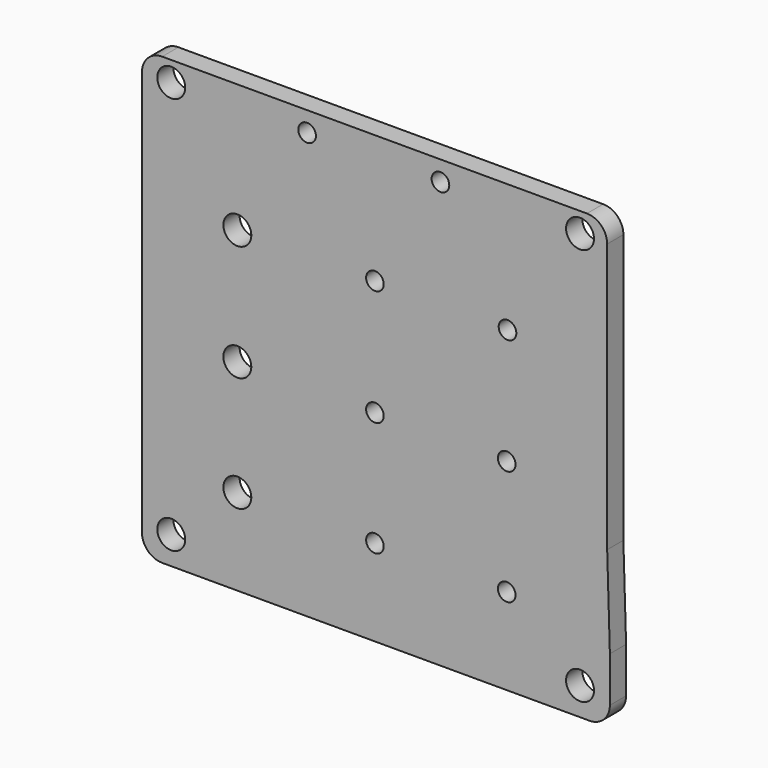
from build123d import *

# Parameters (mm, degrees)
F0_R     = 4.3787819408
F0_R_2   = 2.76225
F1_DEPTH = 6.35


# Not quite as in the source:
# - a feature names something its author has since deleted; it is built from what else it names


with BuildPart() as f1:
    # F0 (on Front) → F1 (new body)
    with BuildSketch(Plane.XZ):
        with BuildLine():
            ThreePointArc((72.7984449517, 70.2034191426), (70.9385730123, 74.6935472031), (66.4484449517, 76.5534191426))
            Line((66.4484449517, 76.5534191426), (-66.6879298329, 76.5534191426))
            ThreePointArc((-66.6879298329, 76.5534191426), (-71.1780578935, 74.6935472031), (-73.0379298329, 70.2034191426))
            Line((-73.0379298329, 70.2034191426), (-73.0379298329, -14.1499808574))
            Line((-73.0379298329, -14.1499808574), (-73.0379298329, -42.5979808574))
            Line((-73.0379298329, -42.5979808574), (-73.0379298329, -56.7965808574))
            ThreePointArc((-73.0379298329, -56.7965808574), (-71.1780578935, -61.286708918), (-66.6879298329, -63.1465808574))
            Line((-66.6879298329, -63.1465808574), (67.2946030807, -63.1465808574))
            ThreePointArc((67.2946030807, -63.1465808574), (71.7847311412, -61.286708918), (73.6446030807, -56.7965808574))
            Line((73.6446030807, -56.7965808574), (73.6446030807, -42.5853939971))
            Line((73.6446030807, -42.5853939971), (72.7984449517, -14.1499808574))
            Line((72.7984449517, -14.1499808574), (72.7984449517, 70.2034191426))
        make_face()
        with Locations((-63.8573840261, -54.3791967528)):
            Circle(F0_R, mode=Mode.SUBTRACT)
        with Locations((-43.1257002056, -36.0373866536)):
            Circle(F0_R, mode=Mode.SUBTRACT)
        with Locations((0, -36.0373866536)):
            Circle(F0_R_2, mode=Mode.SUBTRACT)
        with Locations((-43.1257002056, 0)):
            Circle(F0_R, mode=Mode.SUBTRACT)
        Circle(F0_R_2, mode=Mode.SUBTRACT)
        with Locations((64.2901332332, -54.3791967528)):
            Circle(F0_R, mode=Mode.SUBTRACT)
        with Locations((41.3103699684, -36.0373866536)):
            Circle(F0_R_2, mode=Mode.SUBTRACT)
        with Locations((41.3103699684, 0)):
            Circle(F0_R_2, mode=Mode.SUBTRACT)
        with Locations((-43.1257002056, 36.3284125924)):
            Circle(F0_R, mode=Mode.SUBTRACT)
        with Locations((0, 36.3284125924)):
            Circle(F0_R_2, mode=Mode.SUBTRACT)
        with Locations((-63.8573840261, 70.3177154064)):
            Circle(F0_R, mode=Mode.SUBTRACT)
        with Locations((-21.2588757277, 70.3177154064)):
            Circle(F0_R_2, mode=Mode.SUBTRACT)
        with Locations((41.5558456844, 36.3284125924)):
            Circle(F0_R_2, mode=Mode.SUBTRACT)
        with Locations((20.5344017595, 70.3177154064)):
            Circle(F0_R_2, mode=Mode.SUBTRACT)
        with Locations((64.2901332332, 70.3177154064)):
            Circle(F0_R, mode=Mode.SUBTRACT)
    extrude(amount=F1_DEPTH)


solid = f1.part
